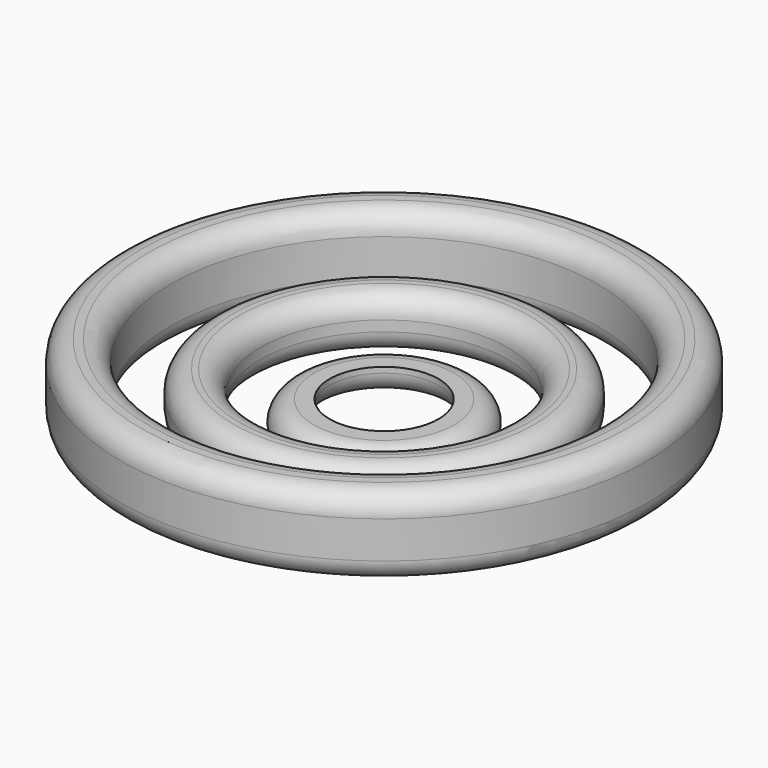
from build123d import *

# Parameters (mm, degrees)
F0_R      = 21.9043363511
F0_R_2    = 13.0604308997
F1_DEPTH  = 6.35
F2_R      = 5.08
F4_R      = 41.1917956684
F4_R_2    = 29.6921655886
F5_DEPTH  = 12.7
F6_R      = 5.08
F7_R      = 5.08
F8_R      = 5.08
F9_R      = 63.3529102605
F9_R_2    = 51.2937601989
F10_DEPTH = 19.05
F11_R     = 5.08
F12_R     = 5.08


# Not quite as in the source:
# - a fillet or chamfer that OpenCascade refuses, or shapes differently, is made with other operations: its cross-section is extruded or revolved along the edge and cut away or added


with BuildPart() as f1:
    # F0 (on Top) → F1 (new body)
    with BuildSketch(Plane.XY):
        Circle(F0_R)
        Circle(F0_R_2, mode=Mode.SUBTRACT)
    extrude(amount=F1_DEPTH)

    # F2
    f2_edges = [f1.edges().sort_by_distance(p)[0] for p in [
        (-21.904336, 0, 6.35),
    ]]
    fillet(f2_edges, radius=F2_R)

    # F3: fillet of radius 5.08 on 2 edges, made by hand

    # F3_s1 → F3_t2 (revolve, cut)
    with BuildSketch(Plane.XZ):
        with BuildLine():
            ThreePointArc((21.9046009047, 1.269699981), (20.3402305458, 0.3277187953), (18.5438672111, -0.0004))
            Line((18.5438672111, -0.0004), (18.5438672111, -0.5085365685))
            ThreePointArc((18.5438672111, -0.5085365685), (20.2241017811, -0.5081365685), (21.9043363511, -0.5081365685))
            Line((21.9043363511, -0.5081365685), (22.4124729197, 0))
            ThreePointArc((22.4124729197, 0), (22.4124729197, 0.6348499905), (22.2406742741, 0.8885734106))
            Line((22.2406742741, 0.8885734106), (21.9046009047, 1.269699981))
        make_face()
    revolve(axis=Axis((0, 0, 0), (0, 0, 1)), mode=Mode.SUBTRACT)

    # F3_s3 → F3_t4 (revolve, cut)
    with BuildSketch(Plane.XZ):
        with BuildLine():
            ThreePointArc((18.1413965851, -0.0004), (14.5483284513, 1.4878975516), (13.0600308997, 5.0809656854))
            Line((13.0600308997, 5.0809656854), (12.5518943312, 5.0809656854))
            ThreePointArc((12.5518943312, 5.0809656854), (12.5522943312, 2.5404828427), (12.5522943312, 0))
            Line((12.5522943312, 0), (13.0604308997, -0.5081365685))
            ThreePointArc((13.0604308997, -0.5081365685), (15.6009137424, -0.5081365685), (18.1413965851, -0.5085365685))
            Line((18.1413965851, -0.5085365685), (18.1413965851, -0.0004))
        make_face()
    revolve(axis=Axis((0, 0, 0), (0, 0, 1)), mode=Mode.SUBTRACT)


with BuildPart() as f5:
    # F4 (on Top) → F5 (new body)
    with BuildSketch(Plane.XY):
        Circle(F4_R)
        Circle(F4_R_2, mode=Mode.SUBTRACT)
    extrude(amount=F5_DEPTH)

    # F6
    f6_edges = [f5.edges().sort_by_distance(p)[0] for p in [
        (-41.191796, 0, 0),
    ]]
    fillet(f6_edges, radius=F6_R)

    # F7
    f7_edges = [f5.edges().sort_by_distance(p)[0] for p in [
        (-29.692166, 0, 0),
    ]]
    fillet(f7_edges, radius=F7_R)

    # F8
    f8_edges = [f5.edges().sort_by_distance(p)[0] for p in [
        (-41.191796, 0, 12.7),
        (-29.692166, 0, 12.7),
    ]]
    fillet(f8_edges, radius=F8_R)


with BuildPart() as f10:
    # F9 (on Top) → F10 (new body)
    with BuildSketch(Plane.XY):
        Circle(F9_R)
        Circle(F9_R_2, mode=Mode.SUBTRACT)
    extrude(amount=F10_DEPTH)

    # F11
    f11_edges = [f10.edges().sort_by_distance(p)[0] for p in [
        (-63.35291, 0, 0),
        (-51.29376, 0, 0),
    ]]
    fillet(f11_edges, radius=F11_R)

    # F12
    f12_edges = [f10.edges().sort_by_distance(p)[0] for p in [
        (-63.35291, 0, 19.05),
        (-51.29376, 0, 19.05),
    ]]
    fillet(f12_edges, radius=F12_R)


solid = Compound([f1.part, f5.part, f10.part])
